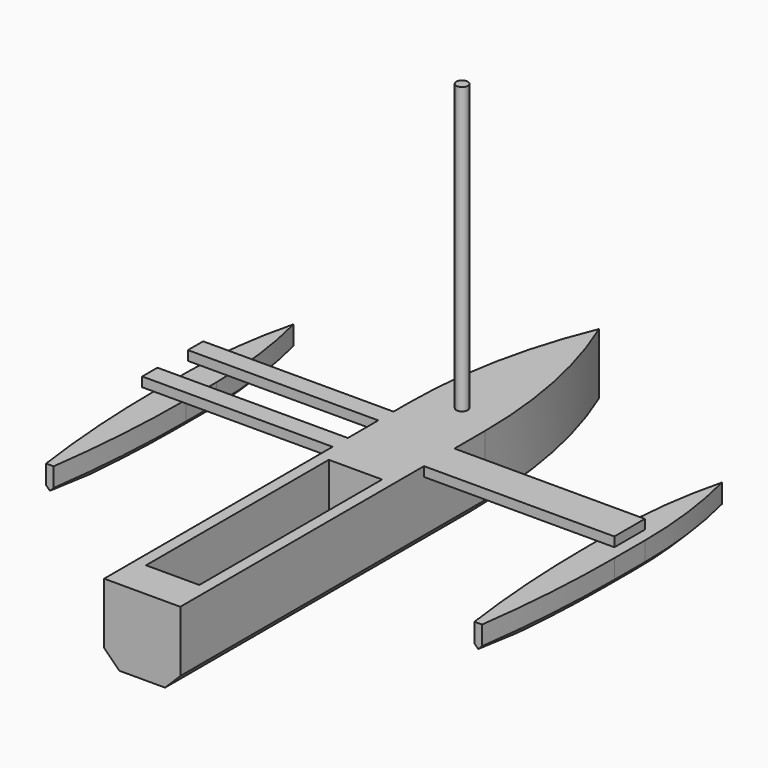
from build123d import *

# Parameters (mm, degrees)
F1_DEPTH    = 400
F3_W        = 1200
F3_H        = 100
F4_DEPTH    = 50
F5_W        = 1000
F5_H        = 200
F6_DEPTH    = 50
F8_START    = -100
F8_DEPTH    = 150
F11_SIZE    = 80
F13_DEPTH   = 300
F14_R       = 30
F15_DEPTH   = 1500
F16_C1_SIZE = 50
F16_C2_SIZE = 49.9996
F17_C1_SIZE = 50
F17_C2_SIZE = 49.9996


# Not quite as in the source:
# - a fillet or chamfer is up to 0.001 mm smaller than in the source, because OpenCascade refuses the exact size


with BuildPart() as f1:
    # F0 (on Top) → F1 (new body)
    with BuildSketch(Plane.XY):
        with BuildLine():
            Line((-200, 0), (0, 0))
            Line((0, 0), (0, 3000))
            ThreePointArc((0, 3000), (-149.5097567964, 2509.9019513593), (-200, 2000))
            Line((-200, 2000), (-200, 0))
        make_face()
    extrude(amount=-F1_DEPTH)

    # F2: F1 across face


with BuildPart() as f1_1:
    add(f1.part)
    add(f1.part.mirror(Plane(origin=(0, 1500, -200), x_dir=(0, 1, 0), z_dir=(1, 0, 0))))

    # F3 (on Top) → F4 (join)
    with BuildSketch(Plane.XY):
        with Locations((-600, 1550)):
            Rectangle(F3_W, F3_H)
        with Locations((-600, 1850)):
            Rectangle(F3_W, F3_H)
    extrude(amount=-F4_DEPTH)

    # F5 (on face) → F6 (join)
    with BuildSketch(Plane.XY):
        with Locations((700, 1700)):
            Rectangle(F5_W, F5_H)
    extrude(amount=-F6_DEPTH)

    # F11
    f11_edges = [f1_1.edges().sort_by_distance(p)[0] for p in [
        (-200, 1000, -400),
        (-149.509757, 2509.901951, -400),
        (149.509757, 2509.901951, -400),
        (200, 1000, -400),
    ]]
    chamfer(f11_edges, length=F11_SIZE)

    # F12 (on face) → F13 (cut)
    with BuildSketch(Plane.XY):
        Polygon((140, 200), (140, 1400), (0, 1400), (-140, 1400), (-140, 200), (0, 200), align=None)
    extrude(amount=-F13_DEPTH, mode=Mode.SUBTRACT)

    # F14 (on face) → F15 (join)
    with BuildSketch(Plane.XY):
        with Locations((0, 2100)):
            Circle(F14_R)
    extrude(amount=F15_DEPTH)


with BuildPart() as f8:
    # F7 (on Top) → F8 (new body)
    with BuildSketch(Plane.XY.offset(F8_START)):
        with BuildLine():
            Line((1200, 1600), (1200, 1800))
            ThreePointArc((1200, 1800), (1181.1773244896, 2102.3346655612), (1125, 2400))
            Line((1125, 2400), (1125, 800))
            Line((1125, 800), (1145, 800))
            ThreePointArc((1145, 800), (1186.2337907259, 1199.0558018876), (1200, 1600))
        make_face()
    extrude(amount=-F8_DEPTH)

    # F9: F8 across face


with BuildPart() as f8_1:
    add(f8.part)
    add(f8.part.mirror(Plane(origin=(1125, 1600, -175), x_dir=(0, -1, 0), z_dir=(-1, 0, 0))))


with BuildPart() as f10_1:
    # F10: instance of F8
    add(f8_1.part.mirror(Plane.YZ))

    # F17: chamfer of 50 on 2 edges, made by hand

    # F17_c1
    f17_c1_edges = [f10_1.edges().sort_by_distance(p)[0] for p in [
        (-1200, 1700, -250),
        (-1181.1773244896, 2102.3346655612, -250),
        (-1186.2337907259, 1199.0558018876, -250),
    ]]
    chamfer(f17_c1_edges, length=F17_C1_SIZE)

    # F17_c2 (size 50 in the source; OpenCascade refuses exactly that, so slightly less here)
    f17_c2_edges = [f10_1.edges().sort_by_distance(p)[0] for p in [
        (-1062.3992616244, 2045.5456347202, -250),
        (-1050, 1700, -250),
        (-1062.4591242566, 1218.5436820583, -250),
    ]]
    chamfer(f17_c2_edges, length=F17_C2_SIZE)


with BuildPart() as f8_2:
    add(f8_1.part)

    # F16: chamfer of 50 on 2 edges, made by hand

    # F16_c1
    f16_c1_edges = [f8_2.edges().sort_by_distance(p)[0] for p in [
        (1200, 1700, -250),
        (1181.1773244896, 2102.3346655612, -250),
        (1186.2337907259, 1199.0558018876, -250),
    ]]
    chamfer(f16_c1_edges, length=F16_C1_SIZE)

    # F16_c2 (size 50 in the source; OpenCascade refuses exactly that, so slightly less here)
    f16_c2_edges = [f8_2.edges().sort_by_distance(p)[0] for p in [
        (1062.3992616244, 2045.5456347202, -250),
        (1050, 1700, -250),
        (1062.4591242566, 1218.5436820583, -250),
    ]]
    chamfer(f16_c2_edges, length=F16_C2_SIZE)


solid = Compound([f1_1.part, f10_1.part, f8_2.part])
